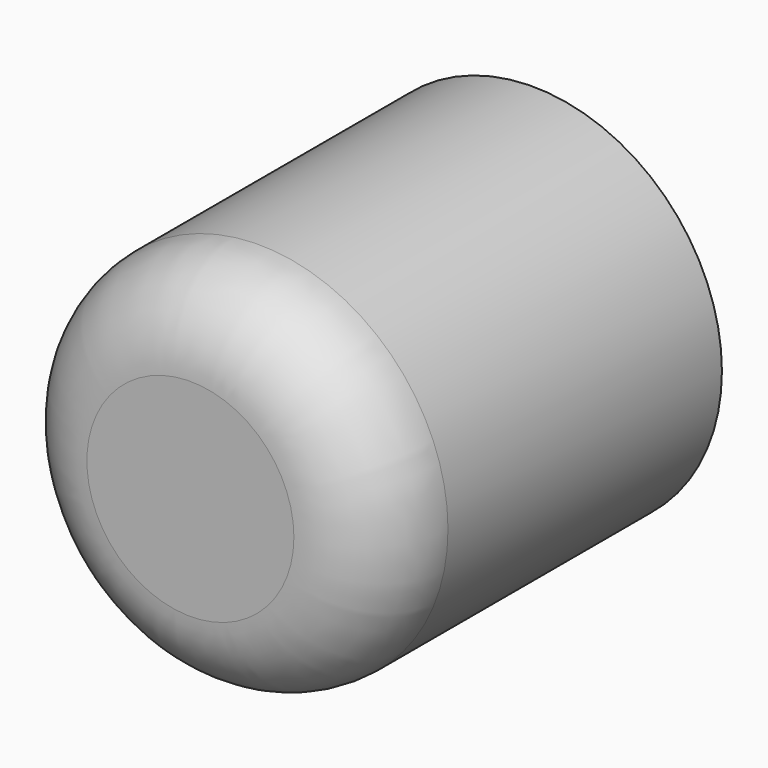
from build123d import *

# Parameters (mm, degrees)
F0_W = 11.223247965
F0_H = 25.4
F2_T = -2.54
F4_R = 5.08


# Not quite as in the source:
# - a fillet or chamfer that OpenCascade refuses, or shapes differently, is made with other operations: its cross-section is extruded or revolved along the edge and cut away or added


with BuildPart() as f1:
    # F0 (on Top) → F1 (revolve)
    with BuildSketch(Plane.XY):
        with Locations((5.6116239825, 12.7)):
            Rectangle(F0_W, F0_H)
    revolve(axis=Axis((0, 12.7, 0), (0, 1, 0)))

    # F2
    f2_openings = [f1.faces().sort_by_distance(p)[0] for p in [
        (0, 25.4, 0),
    ]]
    offset(amount=F2_T, openings=f2_openings)

    # F3: fillet of radius 5.08 on 1 edges, made by hand

    # F3_s1 → F3_t2 (revolve, cut)
    with BuildSketch(Plane.XY):
        with BuildLine():
            ThreePointArc((11.223247965, 25.4), (9.3638389137, 23.5405909488), (8.683247965, 21.0005909488))
            Line((8.683247965, 21.0005909488), (8.581647965, 21.0005909488))
            Line((8.581647965, 21.0005909488), (8.581647965, 25.4))
            Line((8.581647965, 25.4), (8.683247965, 25.5016))
            ThreePointArc((8.683247965, 25.5016), (9.953247965, 25.5016), (11.172447965, 25.487988181))
            Line((11.172447965, 25.487988181), (11.223247965, 25.4))
        make_face()
    revolve(axis=Axis((0, 25.4, 0), (0, 1, 0)), mode=Mode.SUBTRACT)

    # F4
    f4_edges = [f1.edges().sort_by_distance(p)[0] for p in [
        (-11.223248, 0, 0),
    ]]
    fillet(f4_edges, radius=F4_R)


solid = f1.part
